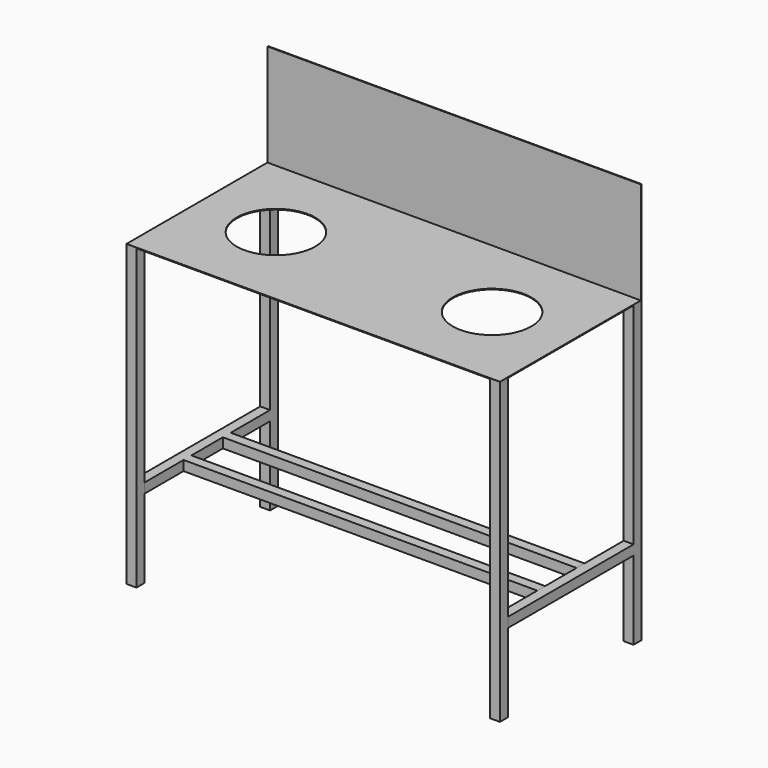
from build123d import *

# Parameters (mm, degrees)
F0_W      = 25
F0_H      = 25
F1_DEPTH  = 760
F2_DEPTH  = 760
F3_W      = 950
F3_H      = 450
F4_DEPTH  = 2
F5_W      = 950
F5_H      = 2
F6_DEPTH  = 260
F7_W      = 25
F7_H      = 25
F8_DEPTH  = 400
F9_W      = 25
F9_H      = 25
F10_DEPTH = 900
F11_R     = 100
F12_DEPTH = 2


with BuildPart() as f1:
    # F0 (on Top) → F1 (new body)
    with BuildSketch(Plane.XY):
        with Locations((-462.5, 212.5)):
            Rectangle(F0_W, F0_H)
    extrude(amount=F1_DEPTH)

    # F3 (on face) → F4 (join)
    with BuildSketch(Plane.XY.offset(760)):
        Rectangle(F3_W, F3_H)
    extrude(amount=F4_DEPTH)

    # F5 (on face) → F6 (join)
    with BuildSketch(Plane.XY.offset(762)):
        with Locations((0, 224)):
            Rectangle(F5_W, F5_H)
    extrude(amount=F6_DEPTH)

    # F7 (on face) → F8 (join, through all)
    with BuildSketch(Plane.XZ.offset(-200)):
        with Locations((-462.5, 212.5)):
            Rectangle(F7_W, F7_H)
    extrude(amount=F8_DEPTH)

    # F9 (on face) → F10 (join)
    with BuildSketch(Plane.YZ.offset(-450)):
        with Locations((62.5, 212.5)):
            Rectangle(F9_W, F9_H)
        with Locations((-62.5, 212.5)):
            Rectangle(F9_W, F9_H)
    extrude(amount=F10_DEPTH)

    # F11 (on face) → F12 (cut, through all)
    with BuildSketch(Plane.XY.offset(762)):
        with Locations((-275, 0)):
            Circle(F11_R)
        with Locations((275, 0)):
            Circle(F11_R)
    extrude(amount=-F12_DEPTH, mode=Mode.SUBTRACT)


with BuildPart() as f2:
    # F0 (on Top) → F2 (new body)
    with BuildSketch(Plane.XY):
        with Locations((462.5, -212.5)):
            Rectangle(F0_W, F0_H)
    extrude(amount=F2_DEPTH)


with BuildPart() as f2b:
    # F0 (on Top) → F2, piece 2 (new body)
    with BuildSketch(Plane.XY):
        with Locations((462.5, 212.5)):
            Rectangle(F0_W, F0_H)
    extrude(amount=F2_DEPTH)

    # F7 (on face) → F8, piece 2 (join, through all)
    with BuildSketch(Plane.XZ.offset(-200)):
        with Locations((462.5, 212.5)):
            Rectangle(F7_W, F7_H)
    extrude(amount=F8_DEPTH)


with BuildPart() as f2c:
    # F0 (on Top) → F2, piece 3 (new body)
    with BuildSketch(Plane.XY):
        with Locations((-462.5, -212.5)):
            Rectangle(F0_W, F0_H)
    extrude(amount=F2_DEPTH)


solid = Compound([f1.part, f2.part, f2b.part, f2c.part])
